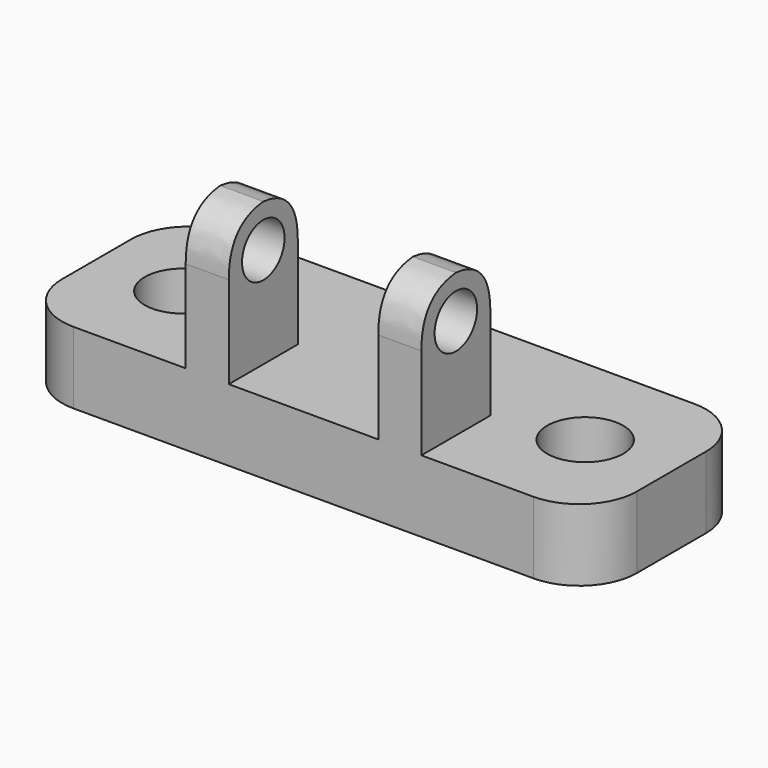
from build123d import *

# Parameters (mm, degrees)
F0_W        = 50.8
F0_H        = 17.78
F0_R        = 3.3655
F1_DEPTH    = 6.35
F2_R        = 5.08
F3_W        = 3.81
F3_H        = 7.62
F4_DEPTH    = 12.7
F5_R        = 2.3495
F6_DEPTH    = 25.4
F7_T1_DEPTH = 26.67
F7_T3_DEPTH = 26.67


# Not quite as in the source:
# - a fillet or chamfer that OpenCascade refuses, or shapes differently, is made with other operations: its cross-section is extruded or revolved along the edge and cut away or added


with BuildPart() as f1:
    # F0 (on Top) → F1 (new body)
    with BuildSketch(Plane.XY):
        with Locations((14.6050021708, -2.1469597467)):
            Rectangle(F0_W, F0_H)
        with Locations((-3.1749978292, -2.1469597467)):
            Circle(F0_R, mode=Mode.SUBTRACT)
        with Locations((32.3850021708, -2.1469597467)):
            Circle(F0_R, mode=Mode.SUBTRACT)
    extrude(amount=F1_DEPTH)

    # F2
    f2_edges = [f1.edges().sort_by_distance(p)[0] for p in [
        (40.005002, -11.03696, 3.175),
        (40.005002, 6.74304, 3.175),
        (-10.794998, -11.03696, 3.175),
        (-10.794998, 6.74304, 3.175),
    ]]
    fillet(f2_edges, radius=F2_R)

    # F3 (on face) → F4 (join)
    with BuildSketch(Plane.XY.offset(6.35)):
        with Locations((6.0960021708, -7.2269597467)):
            Rectangle(F3_W, F3_H)
        with Locations((23.1140021708, -7.2269597467)):
            Rectangle(F3_W, F3_H)
    extrude(amount=F4_DEPTH)

    # F5 (on face) → F6 (cut)
    with BuildSketch(Plane.YZ.offset(25.0190021708)):
        with Locations((-7.2269597467, 15.24)):
            Circle(F5_R)
    extrude(amount=-F6_DEPTH, mode=Mode.SUBTRACT)

    # F7: fillet of radius 4.572 on 4 edges, made by hand

    # F7_s2 → F7_t1 (cut)
    with BuildSketch(Plane.YZ.offset(-7.2389978292)):
        with BuildLine():
            add(Edge.make_bspline(
                [(-11.0369597467, 14.478), (-11.0369597467, 19.05), (-6.4649597467, 19.05)],
                knots=[0, 0, 0, 1, 1, 1], degree=2, weights=[1, 1, 1]))
            Line((-6.4649597467, 19.05), (-11.0369597467, 19.05))
            Line((-11.0369597467, 19.05), (-11.0369597467, 14.478))
        make_face()
        with BuildLine():
            add(Edge.make_bspline(
                [(-3.4169597467, 14.478), (-3.4169597467, 19.05), (-7.9889597467, 19.05)],
                knots=[0, 0, 0, 1, 1, 1], degree=2, weights=[1, 1, 1]))
            Line((-7.9889597467, 19.05), (-3.4169597467, 19.05))
            Line((-3.4169597467, 19.05), (-3.4169597467, 14.478))
        make_face()
    extrude(amount=F7_T1_DEPTH, mode=Mode.SUBTRACT)

    # F7_s4 → F7_t3 (cut)
    with BuildSketch(Plane.YZ.offset(9.7790021708)):
        with BuildLine():
            add(Edge.make_bspline(
                [(-11.0369597467, 14.478), (-11.0369597467, 19.05), (-6.4649597467, 19.05)],
                knots=[0, 0, 0, 1, 1, 1], degree=2, weights=[1, 1, 1]))
            Line((-6.4649597467, 19.05), (-11.0369597467, 19.05))
            Line((-11.0369597467, 19.05), (-11.0369597467, 14.478))
        make_face()
        with BuildLine():
            add(Edge.make_bspline(
                [(-3.4169597467, 14.478), (-3.4169597467, 19.05), (-7.9889597467, 19.05)],
                knots=[0, 0, 0, 1, 1, 1], degree=2, weights=[1, 1, 1]))
            Line((-7.9889597467, 19.05), (-3.4169597467, 19.05))
            Line((-3.4169597467, 19.05), (-3.4169597467, 14.478))
        make_face()
    extrude(amount=F7_T3_DEPTH, mode=Mode.SUBTRACT)


solid = f1.part
